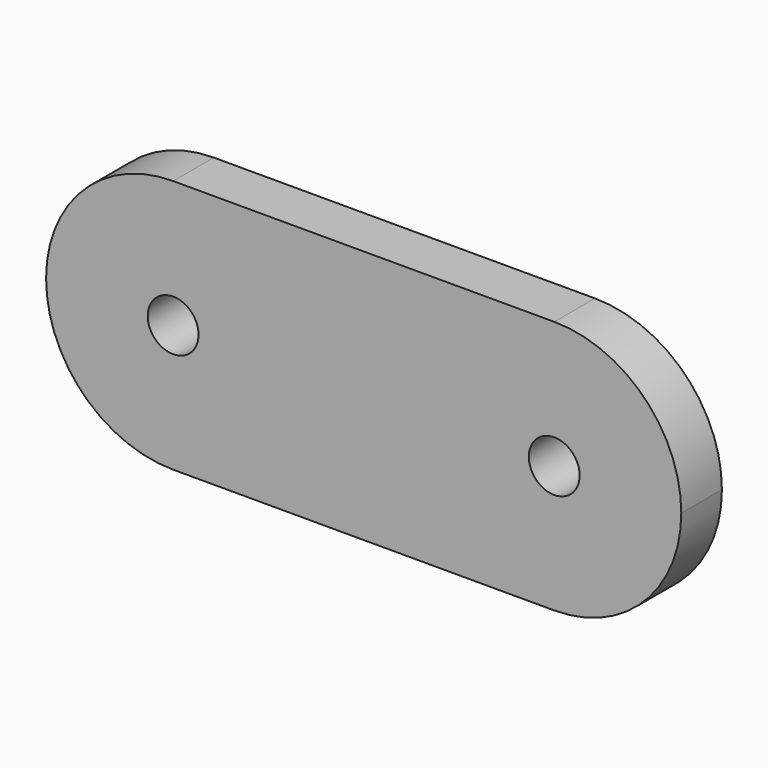
from build123d import *

# Parameters (mm, degrees)
F0_W     = 25
F0_H     = 10
F0_R     = 1
F1_DEPTH = 2
F2_R     = 4.99999


# Not quite as in the source:
# - a fillet or chamfer is up to 0.001 mm smaller than in the source, because OpenCascade refuses the exact size


with BuildPart() as f1:
    # F0 (on Front) → F1 (new body)
    with BuildSketch(Plane.XZ):
        with Locations((12.5, -5)):
            Rectangle(F0_W, F0_H)
        with Locations((5, -5)):
            Circle(F0_R, mode=Mode.SUBTRACT)
        with Locations((20, -5)):
            Circle(F0_R, mode=Mode.SUBTRACT)
    extrude(amount=F1_DEPTH)

    # F2 (radius 5 in the source; OpenCascade refuses exactly that, so slightly less here)
    f2_edges = [f1.edges().sort_by_distance(p)[0] for p in [
        (0, -1, 0),
        (0, -1, -10),
        (25, -1, 0),
        (25, -1, -10),
    ]]
    fillet(f2_edges, radius=F2_R)


solid = f1.part
